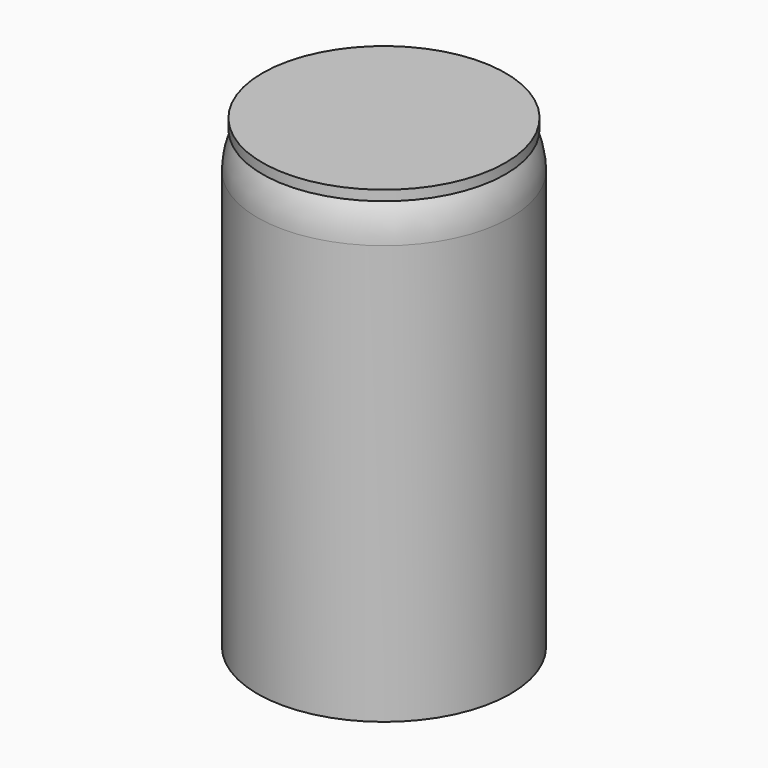
from build123d import *

# Parameters (mm, degrees)
F0_R     = 12.5
F1_DEPTH = 45
F3_R     = 11.5
F3_R_2   = 6.5
F4_DEPTH = 44.5
F2_R     = 6.5
F6_DEPTH = 44.5
F7_R     = 12
F8_DEPTH = 1


# Not quite as in the source:
# - a fillet or chamfer that OpenCascade refuses, or shapes differently, is made with other operations: its cross-section is extruded or revolved along the edge and cut away or added


with BuildPart() as f1:
    # F0 (on Top) → F1 (new body)
    with BuildSketch(Plane.XY):
        Circle(F0_R)
    extrude(amount=F1_DEPTH)

    # F3 (on face) → F4 (cut)
    with BuildSketch(Plane.XY.offset(45)):
        Circle(F3_R)
        Circle(F3_R_2, mode=Mode.SUBTRACT)
    extrude(amount=-F4_DEPTH, mode=Mode.SUBTRACT)

    # F5: fillet of radius 7 on 1 edges, made by hand

    # F5_s1 → F5_t2 (revolve, cut)
    with BuildSketch(Plane.XZ):
        with BuildLine():
            ThreePointArc((12.5, 41.3944487245), (12.2453687816, 43.2652774179), (11.5, 45))
            Line((11.5, 45), (12.5, 45))
            Line((12.5, 45), (12.5, 41.3944487245))
        make_face()
    revolve(axis=Axis((0, 0, 45), (0, 0, 1)), mode=Mode.SUBTRACT)

    # F2 (on face) → F6 (cut)
    with BuildSketch(Plane.XY.offset(45)):
        Circle(F2_R)
    extrude(amount=-F6_DEPTH, mode=Mode.SUBTRACT)


with BuildPart() as f8:
    # F7 (on face) → F8 (new body)
    with BuildSketch(Plane.XY.offset(45)):
        Circle(F7_R)
    extrude(amount=F8_DEPTH)


solid = Compound([f1.part, f8.part])
